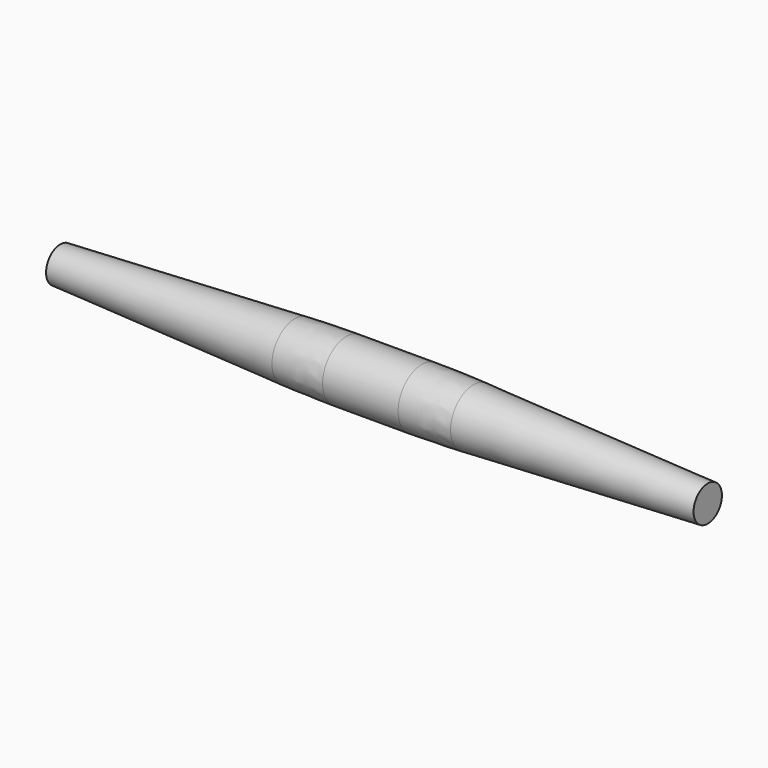
from build123d import *


# Not quite as in the source:
# - a fillet or chamfer that OpenCascade refuses, or shapes differently, is made with other operations: its cross-section is extruded or revolved along the edge and cut away or added


with BuildPart() as f1:
    # F0 (on Front) → F1 (revolve)
    with BuildSketch(Plane.XZ):
        Polygon((0, 9.525), (0, 0), (347.6625, 0), (347.6625, 9.525), (207.9625, 15.875), (139.7, 15.875), align=None)
    revolve(axis=Axis((173.83125, 0, 0), (1, 0, 0)))

    # F2: fillet of radius 609.6 on 2 edges, made by hand

    # F2_s1 → F2_t2 (revolve, cut)
    with BuildSketch(Plane.XZ):
        with BuildLine():
            ThreePointArc((153.5473965644, 15.875), (139.7035712187, 15.7177852553), (125.8668864684, 15.2462221122))
            Line((125.8668864684, 15.2462221122), (139.7, 15.875))
            Line((139.7, 15.875), (153.5473965644, 15.875))
        make_face()
    revolve(axis=Axis((139.7, 0, 0), (1, 0, 0)), mode=Mode.SUBTRACT)

    # F2_s3 → F2_t4 (revolve, cut)
    with BuildSketch(Plane.XZ):
        with BuildLine():
            ThreePointArc((221.7956135316, 15.2462221122), (207.9589287813, 15.7177852553), (194.1151034356, 15.875))
            Line((194.1151034356, 15.875), (207.9625, 15.875))
            Line((207.9625, 15.875), (221.7956135316, 15.2462221122))
        make_face()
    revolve(axis=Axis((207.9625, 0, 0), (1, 0, 0)), mode=Mode.SUBTRACT)


solid = f1.part
